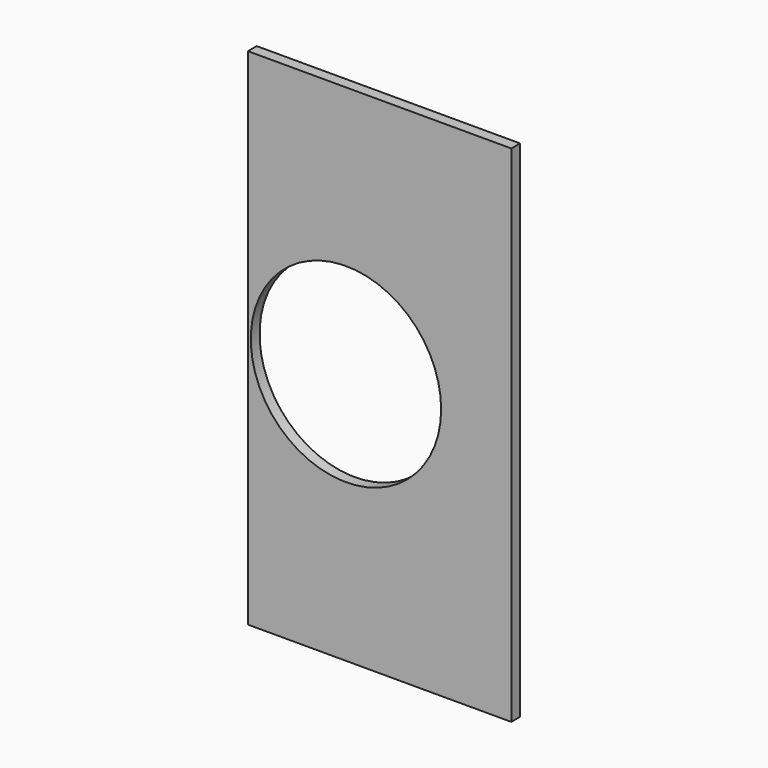
from build123d import *

# Parameters (mm, degrees)
F0_W     = 38.1
F0_H     = 73.025
F1_DEPTH = 1.5875
F2_R     = 13.7668
F3_DEPTH = 25.4


# Not quite as in the source:
# - a length typed as a fraction of an inch, garbled in the dataset ("3 / 203.2 mm" for 3/8 in), is restored


with BuildPart() as f1:
    # F0 (on Front) → F1 (new body)
    with BuildSketch(Plane.XZ):
        Rectangle(F0_W, F0_H)
    extrude(amount=F1_DEPTH)

    # F2 (on face) → F3 (cut)
    with BuildSketch(Plane.XZ.offset(1.5875)):
        with Locations((-4.8653118451, 0)):
            Circle(F2_R)
    extrude(amount=-F3_DEPTH, mode=Mode.SUBTRACT)


solid = f1.part
